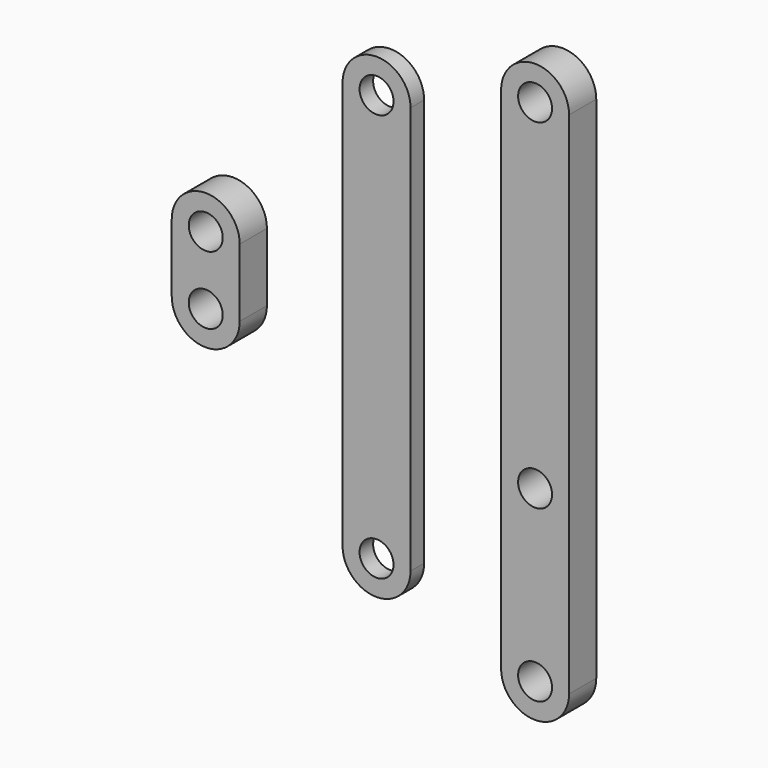
from build123d import *

# Parameters (mm, degrees)
F0_R     = 2.5
F1_DEPTH = 2.5
F2_R     = 2.5
F3_DEPTH = 1.25
F4_R     = 2.5
F5_DEPTH = 2.5


# Not quite as in the source:
# - a feature names something its author has since deleted; it is built from what else it names


with BuildPart() as f1:
    # F0 (on Front) → F1 (new body, symmetric)
    with BuildSketch(Plane.XZ):
        with BuildLine():
            Line((5, 0), (5, 37.5))
            ThreePointArc((5, 37.5), (0, 42.5), (-5, 37.5))
            Line((-5, 37.5), (-5, 0))
            Line((-5, 0), (-5, -37.5))
            ThreePointArc((-5, -37.5), (0, -42.5), (5, -37.5))
            Line((5, -37.5), (5, 0))
        make_face()
        with Locations((0, -37.5)):
            Circle(F0_R, mode=Mode.SUBTRACT)
        with Locations((0, -12.5)):
            Circle(F0_R, mode=Mode.SUBTRACT)
        with Locations((0, 37.5)):
            Circle(F0_R, mode=Mode.SUBTRACT)
    extrude(amount=F1_DEPTH, both=True)


with BuildPart() as f3:
    # F2 (on Front) → F3 (new body, symmetric)
    with BuildSketch(Plane.XZ):
        with BuildLine():
            Line((-19.3265285343, 0), (-19.3265285343, 30))
            ThreePointArc((-19.3265285343, 30), (-24.3265285343, 35), (-29.3265285343, 30))
            Line((-29.3265285343, 30), (-29.3265285343, 0))
            Line((-29.3265285343, 0), (-29.3265285343, -30))
            ThreePointArc((-29.3265285343, -30), (-24.3265285343, -35), (-19.3265285343, -30))
            Line((-19.3265285343, -30), (-19.3265285343, 0))
        make_face()
        with Locations((-24.3265285343, -30)):
            Circle(F2_R, mode=Mode.SUBTRACT)
        with Locations((-24.3265285343, 30)):
            Circle(F2_R, mode=Mode.SUBTRACT)
    extrude(amount=F3_DEPTH, both=True)


with BuildPart() as f5:
    # F4 (on Front) → F5 (new body, symmetric)
    with BuildSketch(Plane.XZ):
        with BuildLine():
            Line((-43.4575378895, 0), (-43.4575378895, 5))
            ThreePointArc((-43.4575378895, 5), (-48.4575378895, 10), (-53.4575378895, 5))
            Line((-53.4575378895, 5), (-53.4575378895, 0))
            Line((-53.4575378895, 0), (-53.4575378895, -5))
            ThreePointArc((-53.4575378895, -5), (-48.4575378895, -10), (-43.4575378895, -5))
            Line((-43.4575378895, -5), (-43.4575378895, 0))
        make_face()
        with Locations((-48.4575378895, -5)):
            Circle(F4_R, mode=Mode.SUBTRACT)
        with Locations((-48.4575378895, 5)):
            Circle(F4_R, mode=Mode.SUBTRACT)
    extrude(amount=F5_DEPTH, both=True)


solid = Compound([f1.part, f3.part, f5.part])
